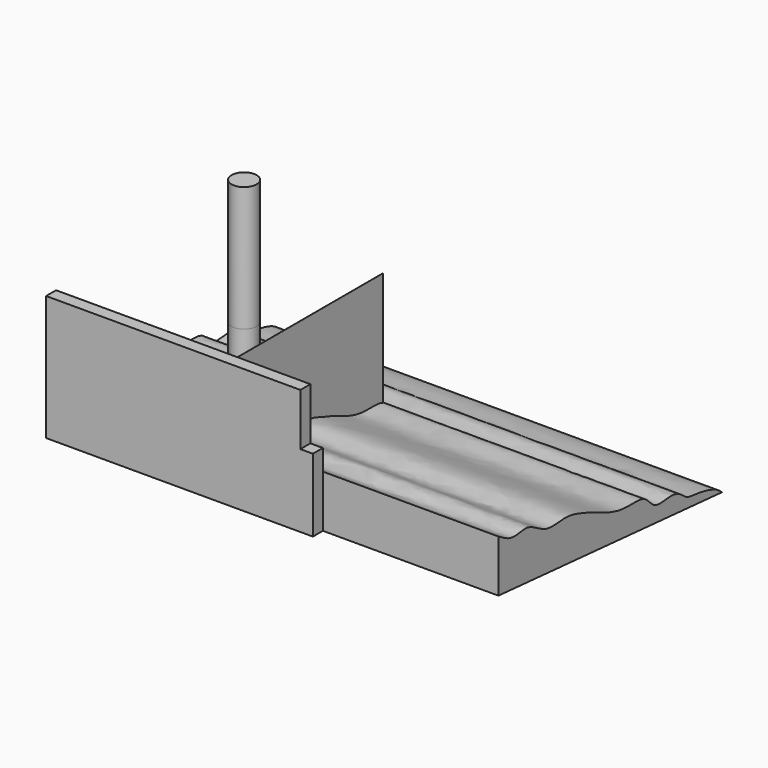
from build123d import *

# Parameters (mm, degrees)
F0_W      = 5800
F0_H      = 300
F1_DEPTH  = 3000
F2_W      = 300
F2_H      = 1750
F3_DEPTH  = 300
F4_W      = 300
F4_H      = 1960
F4_H_2    = 1040
F5_DEPTH  = 300
F12_DEPTH = 10610
F11_R     = 300
F14_DEPTH = 3000
F10_E8_W  = 3000
F10_E8_H  = 4360
F15_DEPTH = 1


# Not quite as in the source:
# - a feature of the source that left no trace in its solid (it failed there, or was rolled back) is left out


with BuildPart() as f1:
    # F0 (on Top) → F1 (new body)
    with BuildSketch(Plane.XY):
        with Locations((2900, -150)):
            Rectangle(F0_W, F0_H)
    extrude(amount=F1_DEPTH)

    # F2 (on face) → F3 (join)
    with BuildSketch(Plane.YZ.offset(5800)):
        with Locations((-150, 875)):
            Rectangle(F2_W, F2_H)
    extrude(amount=F3_DEPTH)

    # F4 (on face) → F5 (join)
    with BuildSketch(Plane(origin=(0, 0, 0), x_dir=(0, -1, 0), z_dir=(-1, 0, 0))):
        with Locations((150, 980)):
            Rectangle(F4_W, F4_H)
        with Locations((150, 2480)):
            Rectangle(F4_W, F4_H_2)
    extrude(amount=F5_DEPTH)


with BuildPart() as f12:
    # F8 (on face) → F12 (new body)
    with BuildSketch(Plane(origin=(-300, 0, 0), x_dir=(0, -1, 0), z_dir=(-1, 0, 0))):
        with BuildLine():
            Line((0, 0), (0, 1250))
            add(Edge.make_bspline(
                [(0, 1250), (-143.1748461176, 1160.4540186162), (-426.5021162652, 983.2523721949), (-917.1022397172, 1181.3960526208), (-1406.5603052218, 729.6623883693), (-1981.6866568889, 871.1262336875), (-2428.3239658637, 760.8439284346), (-2942.5940967446, 567.2961590142), (-3680.9226802544, 234.724526235), (-4417.1426534692, 380.6415969382), (-4655.0024542936, -113.7698280504), (-5218.2226437508, 64.2754910253), (-5526.2709066711, -109.4112998292), (-5646.3793917658, -247.3628347645), (-6026.2768963987, -257.3225241521), (-6517.1710983426, -379.1301511217), (-6648.8150937925, -494.1101038226), (-6701.7860412598, -540.3757691383)],
                knots=[0, 0, 0, 0, 0.068075911, 0.1347147389, 0.2102598907, 0.2834803393, 0.3491753838, 0.422133231, 0.511304785, 0.5918912576, 0.6553500627, 0.7260005804, 0.7824312848, 0.8223100383, 0.8819426474, 0.9524960497, 1, 1, 1, 1], degree=3))
            Line((-6701.7860412598, -540.3757691383), (0, 0))
        make_face()
    extrude(amount=-F12_DEPTH)

    # F11 (on face) → F13 (join, up to the next surface of F12)
    with BuildSketch(Plane.XY.offset(3000)):
        with Locations((3250, 1200)):
            Circle(F11_R)
    extrude(until=Until.NEXT, dir=(0, 0, -1))

    # F14 (add): a face of the model
    f14_faces = [f12.faces().sort_by_distance(p)[0] for p in [
        (3250, 1200, 3000),
    ]]
    extrude(f14_faces, amount=F14_DEPTH)


with BuildPart() as f15:
    # F10_E8 (on explicit) → F15 (new body)
    with BuildSketch(Plane(origin=(4050, 0, 3000), x_dir=(0, 0, -1), z_dir=(1, 0, 0))):
        with Locations((1500, 2180)):
            Rectangle(F10_E8_W, F10_E8_H)
    extrude(amount=F15_DEPTH)


solid = Compound([f1.part, f12.part, f15.part])
